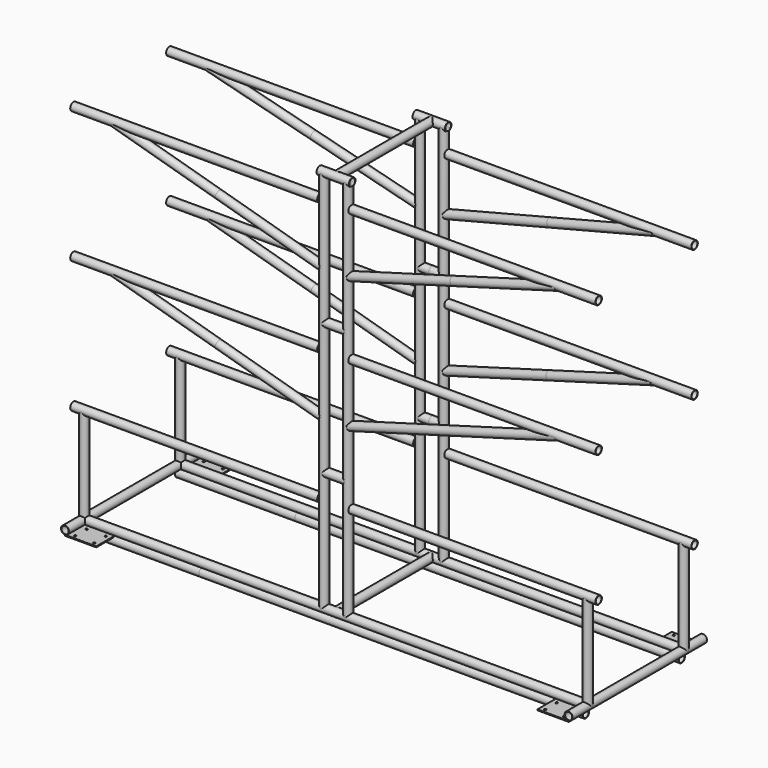
from build123d import *

# Parameters (mm, degrees)
F1_DEPTH       = 1600
F3_R           = 17
F4_DEPTH       = 50
F4_DEPTH_BACK  = 650
F5_DEPTH       = 50
F5_DEPTH_BACK  = 650
F7_R           = 17
F8_DEPTH       = 500
F8_DEPTH_BACK  = 1600
F10_W          = 130
F10_H          = 100
F10_R          = 4.5
F11_DEPTH      = 4
F14_R          = 17
F15_DEPTH      = 500
F15_DEPTH_BACK = 1600
F17_R          = 17
F18_DEPTH      = 500
F21_R          = 17
F22_DEPTH      = 530
F22_DEPTH_BACK = 500
F24_R          = 17
F25_DEPTH      = 530
F25_DEPTH_BACK = 500
F27_R          = 17
F28_DEPTH      = 450
F28_DEPTH_BACK = 450
F30_R          = 17
F31_DEPTH      = 450
F31_DEPTH_BACK = 450
F33_R          = 17
F34_DEPTH      = 50
F34_DEPTH_BACK = 50
F35_DEPTH      = 67.5
F35_DEPTH_BACK = 67.5
F37_R          = 17
F38_DEPTH      = 450
F38_DEPTH_BACK = 450
F40_R          = 17
F41_DEPTH      = 450
F41_DEPTH_BACK = 450
F45_R          = 17
F46_DEPTH      = 530
F46_DEPTH_BACK = 500
F48_R          = 17
F49_DEPTH      = 530
F49_DEPTH_BACK = 500
F51_R          = 17
F52_DEPTH      = 450
F52_DEPTH_BACK = 450
F54_R          = 17
F55_DEPTH      = 450
F55_DEPTH_BACK = 450
F57_R          = 17
F58_DEPTH      = 50
F58_DEPTH_BACK = 50
F59_DEPTH      = 67.5
F59_DEPTH_BACK = 67.5
F61_R          = 17
F62_DEPTH      = 450
F62_DEPTH_BACK = 450
F64_R          = 17
F65_DEPTH      = 450
F65_DEPTH_BACK = 450
F67_R          = 17
F68_DEPTH      = 200
F68_DEPTH_BACK = 200
F67_R_2        = 17.5
F70_R          = 17
F71_DEPTH      = 500
F72_R          = 15
F73_DEPTH      = 1020
F74_R          = 15
F75_DEPTH      = 1020
F76_R          = 15
F77_DEPTH      = 1020
F78_R          = 15
F79_DEPTH      = 1020
F80_R          = 15
F81_DEPTH      = 1020
F82_R          = 15
F83_DEPTH      = 1020
F84_R          = 15
F85_DEPTH      = 200
F86_R          = 15
F87_DEPTH      = 200
F88_R          = 15
F89_DEPTH      = 1020
F90_R          = 15
F91_DEPTH      = 1020
F92_R          = 15
F93_DEPTH      = 1020
F94_R          = 15
F95_DEPTH      = 1020
F96_R          = 15
F97_DEPTH      = 1020
F98_R          = 15
F99_DEPTH      = 1020
F100_R         = 15
F101_DEPTH     = 2300
F102_R         = 15
F103_DEPTH     = 2300
F104_R         = 15
F105_DEPTH     = 700
F106_R         = 15
F107_DEPTH     = 700


with BuildPart() as f1:
    # F0 (on Top) → F1 (new body)
    with BuildSketch(Plane.XY):
        with BuildLine():
            ThreePointArc((-25.1075440943, -100), (-42.1075440943, -83), (-59.1075440943, -100))
            ThreePointArc((-59.1075440943, -100), (-42.1075440943, -117), (-25.1075440943, -100))
        make_face()
    extrude(amount=F1_DEPTH)

    # F45 (on line) → F46 (join, two sides)
    with BuildSketch(Plane(origin=(-557.1075440943, 0, 0), x_dir=(0, -1, 0), z_dir=(-1, 0, 0))) as f46_sk:
        with Locations((100, 1500)):
            Circle(F45_R)
        with Locations((100, 950)):
            Circle(F45_R)
        with Locations((100, 400)):
            Circle(F45_R)
    extrude(amount=F46_DEPTH)
    extrude(f46_sk.sketch, amount=-F46_DEPTH_BACK)

    # F51 (on line) → F52 (join, two sides)
    with BuildSketch(Plane(origin=(-662.975364018, 0, 188.3452738687), x_dir=(0, -1, 0), z_dir=(-0.9619353575, 0, 0.2732770902))) as f52_sk:
        with Locations((100, 661.8477231125)):
            Circle(F51_R)
    extrude(amount=F52_DEPTH)
    extrude(f52_sk.sketch, amount=-F52_DEPTH_BACK)

    # F57 (on line) → F58 (join, two sides)
    with BuildSketch(Plane(origin=(7.8924559057, 0, 0), x_dir=(0, -1, 0), z_dir=(-1, 0, 0))) as f58_sk:
        with Locations((100, 1050)):
            Circle(F57_R)
        with Locations((100, 500)):
            Circle(F57_R)
    extrude(amount=F58_DEPTH)
    extrude(f58_sk.sketch, amount=-F58_DEPTH_BACK)

    # F61 (on line) → F62 (join, two sides)
    with BuildSketch(Plane(origin=(-787.0224706544, 0, 199.8620659412), x_dir=(0, -1, 0), z_dir=(-0.9692356631, 0, 0.2461345759))) as f62_sk:
        with Locations((100, 1225.2471397676)):
            Circle(F61_R)
    extrude(amount=F62_DEPTH)
    extrude(f62_sk.sketch, amount=-F62_DEPTH_BACK)


with BuildPart() as f1b:
    # F0 (on Top) → F1, piece 2 (new body)
    with BuildSketch(Plane.XY):
        with BuildLine():
            ThreePointArc((74.8924559057, -100), (57.8924559057, -83), (40.8924559057, -100))
            ThreePointArc((40.8924559057, -100), (57.8924559057, -117), (74.8924559057, -100))
        make_face()
    extrude(amount=F1_DEPTH)

    # F48 (on line) → F49 (join, two sides)
    with BuildSketch(Plane.YZ.offset(572.8924559057)) as f49_sk:
        with Locations((-100, 1500)):
            Circle(F48_R)
        with Locations((-100, 950)):
            Circle(F48_R)
        with Locations((-100, 400)):
            Circle(F48_R)
    extrude(amount=F49_DEPTH)
    extrude(f49_sk.sketch, amount=-F49_DEPTH_BACK)

    # F54 (on line) → F55 (join, two sides)
    with BuildSketch(Plane(origin=(677.581452806, 0, 192.4947309108), x_dir=(0, 1, 0), z_dir=(0.9619353575, 0, 0.2732770902))) as f55_sk:
        with Locations((-100, 657.5340683437)):
            Circle(F54_R)
    extrude(amount=F55_DEPTH)
    extrude(f55_sk.sketch, amount=-F55_DEPTH_BACK)

    # F64 (on line) → F65 (join, two sides)
    with BuildSketch(Plane(origin=(801.8510973168, 0, 203.6277525262), x_dir=(0, 1, 0), z_dir=(0.9692356631, 0, 0.2461345759))) as f65_sk:
        with Locations((-100, 1221.361927194)):
            Circle(F64_R)
    extrude(amount=F65_DEPTH)
    extrude(f65_sk.sketch, amount=-F65_DEPTH_BACK)


with BuildPart() as f1c:
    # F0 (on Top) → F1, piece 3 (new body)
    with BuildSketch(Plane.XY):
        with BuildLine():
            ThreePointArc((-25.1075440943, -600), (-42.1075440943, -583), (-59.1075440943, -600))
            ThreePointArc((-59.1075440943, -600), (-42.1075440943, -617), (-25.1075440943, -600))
        make_face()
    extrude(amount=F1_DEPTH)

    # F24 (on line) → F25 (join, two sides)
    with BuildSketch(Plane(origin=(-557.1075440943, 0, 0), x_dir=(0, -1, 0), z_dir=(-1, 0, 0))) as f25_sk:
        with Locations((600, 1500)):
            Circle(F24_R)
        with Locations((600, 950)):
            Circle(F24_R)
        with Locations((600, 400)):
            Circle(F24_R)
    extrude(amount=F25_DEPTH)
    extrude(f25_sk.sketch, amount=-F25_DEPTH_BACK)

    # F30 (on line) → F31 (join, two sides)
    with BuildSketch(Plane(origin=(-807.5565565141, 0, 229.4194762824), x_dir=(0, -1, 0), z_dir=(-0.9619353575, 0, 0.2732770902))) as f31_sk:
        with Locations((600, 1190.9121697279)):
            Circle(F30_R)
    extrude(amount=F31_DEPTH)
    extrude(f31_sk.sketch, amount=-F31_DEPTH_BACK)

    # F40 (on line) → F41 (join, two sides)
    with BuildSketch(Plane(origin=(-662.975364018, 0, 188.3452738687), x_dir=(0, -1, 0), z_dir=(-0.9619353575, 0, 0.2732770902))) as f41_sk:
        with Locations((600, 661.8477231125)):
            Circle(F40_R)
    extrude(amount=F41_DEPTH)
    extrude(f41_sk.sketch, amount=-F41_DEPTH_BACK)


with BuildPart() as f1d:
    # F0 (on Top) → F1, piece 4 (new body)
    with BuildSketch(Plane.XY):
        with BuildLine():
            ThreePointArc((74.8924559057, -600), (57.8924559057, -583), (40.8924559057, -600))
            ThreePointArc((40.8924559057, -600), (57.8924559057, -617), (74.8924559057, -600))
        make_face()
    extrude(amount=F1_DEPTH)

    # F21 (on line) → F22 (join, two sides)
    with BuildSketch(Plane.YZ.offset(572.8924559057)) as f22_sk:
        with Locations((-600, 1500)):
            Circle(F21_R)
        with Locations((-600, 950)):
            Circle(F21_R)
        with Locations((-600, 400)):
            Circle(F21_R)
    extrude(amount=F22_DEPTH)
    extrude(f22_sk.sketch, amount=-F22_DEPTH_BACK)

    # F27 (on line) → F28 (join, two sides)
    with BuildSketch(Plane(origin=(822.1626453021, 0, 233.5689333245), x_dir=(0, 1, 0), z_dir=(0.9619353575, 0, 0.2732770902))) as f28_sk:
        with Locations((-600, 1186.5985149591)):
            Circle(F27_R)
    extrude(amount=F28_DEPTH)
    extrude(f28_sk.sketch, amount=-F28_DEPTH_BACK)


with BuildPart() as f4:
    # F3 (on line) → F4 (new body, two sides)
    with BuildSketch(Plane(origin=(0, -50, 0), x_dir=(-1, 0, 0), z_dir=(0, 1, 0))) as f4_sk:
        with Locations((1042.1075440943, 0)):
            Circle(F3_R)
    extrude(amount=F4_DEPTH)
    extrude(f4_sk.sketch, amount=-F4_DEPTH_BACK)


with BuildPart() as f4b:
    # F3 (on line) → F4, piece 2 (new body, two sides)
    with BuildSketch(Plane(origin=(0, -50, 0), x_dir=(-1, 0, 0), z_dir=(0, 1, 0))) as f4_2_sk:
        with Locations((-1057.8924559057, 0)):
            Circle(F3_R)
    extrude(amount=F4_DEPTH)
    extrude(f4_2_sk.sketch, amount=-F4_DEPTH_BACK)


with BuildPart() as f5:
    # F3 (on line) → F5 (new body, two sides)
    with BuildSketch(Plane(origin=(0, -50, 0), x_dir=(-1, 0, 0), z_dir=(0, 1, 0))) as f5_sk:
        with Locations((1042.1075440943, 0)):
            Circle(F3_R)
    extrude(amount=F5_DEPTH)
    extrude(f5_sk.sketch, amount=-F5_DEPTH_BACK)


with BuildPart() as f5b:
    # F3 (on line) → F5, piece 2 (new body, two sides)
    with BuildSketch(Plane(origin=(0, -50, 0), x_dir=(-1, 0, 0), z_dir=(0, 1, 0))) as f5_2_sk:
        with Locations((-1057.8924559057, 0)):
            Circle(F3_R)
    extrude(amount=F5_DEPTH)
    extrude(f5_2_sk.sketch, amount=-F5_DEPTH_BACK)


with BuildPart() as f8:
    # F7 (on line) → F8 (new body, two sides)
    with BuildSketch(Plane.YZ.offset(-550.6075440943)) as f8_sk:
        with Locations((-100, 0)):
            Circle(F7_R)
    extrude(amount=-F8_DEPTH)
    extrude(f8_sk.sketch, amount=F8_DEPTH_BACK)


with BuildPart() as f8b:
    # F7 (on line) → F8, piece 2 (new body, two sides)
    with BuildSketch(Plane.YZ.offset(-550.6075440943)) as f8_2_sk:
        with Locations((-600, 0)):
            Circle(F7_R)
    extrude(amount=-F8_DEPTH)
    extrude(f8_2_sk.sketch, amount=F8_DEPTH_BACK)


with BuildPart() as f11:
    # F10 (on offset) → F11 (new body)
    with BuildSketch(Plane.XY.offset(-17.5)):
        with Locations((-977.1075440943, -650)):
            Rectangle(F10_W, F10_H)
        with Locations((-1012.1075440943, -685)):
            Circle(F10_R, mode=Mode.SUBTRACT)
        with Locations((-932.1075440943, -685)):
            Circle(F10_R, mode=Mode.SUBTRACT)
        with Locations((-1012.1075440943, -625)):
            Circle(F10_R, mode=Mode.SUBTRACT)
        with Locations((-932.1075440943, -625)):
            Circle(F10_R, mode=Mode.SUBTRACT)
    extrude(amount=-F11_DEPTH)


with BuildPart() as f11b:
    # F10 (on offset) → F11, piece 2 (new body)
    with BuildSketch(Plane.XY.offset(-17.5)):
        with Locations((-977.1075440943, -50)):
            Rectangle(F10_W, F10_H)
        with Locations((-1012.1075440943, -75)):
            Circle(F10_R, mode=Mode.SUBTRACT)
        with Locations((-932.1075440943, -75)):
            Circle(F10_R, mode=Mode.SUBTRACT)
        with Locations((-1012.1075440943, -15)):
            Circle(F10_R, mode=Mode.SUBTRACT)
        with Locations((-932.1075440943, -15)):
            Circle(F10_R, mode=Mode.SUBTRACT)
    extrude(amount=-F11_DEPTH)


with BuildPart() as f11c:
    # F10 (on offset) → F11, piece 3 (new body)
    with BuildSketch(Plane.XY.offset(-17.5)):
        with Locations((992.8924559057, -650)):
            Rectangle(F10_W, F10_H)
        with Locations((947.8924559057, -685)):
            Circle(F10_R, mode=Mode.SUBTRACT)
        with Locations((1027.8924559057, -685)):
            Circle(F10_R, mode=Mode.SUBTRACT)
        with Locations((947.8924559057, -625)):
            Circle(F10_R, mode=Mode.SUBTRACT)
        with Locations((1027.8924559057, -625)):
            Circle(F10_R, mode=Mode.SUBTRACT)
    extrude(amount=-F11_DEPTH)


with BuildPart() as f11d:
    # F10 (on offset) → F11, piece 4 (new body)
    with BuildSketch(Plane.XY.offset(-17.5)):
        with Locations((992.8924559057, -50)):
            Rectangle(F10_W, F10_H)
        with Locations((947.8924559057, -75)):
            Circle(F10_R, mode=Mode.SUBTRACT)
        with Locations((1027.8924559057, -75)):
            Circle(F10_R, mode=Mode.SUBTRACT)
        with Locations((947.8924559057, -15)):
            Circle(F10_R, mode=Mode.SUBTRACT)
        with Locations((1027.8924559057, -15)):
            Circle(F10_R, mode=Mode.SUBTRACT)
    extrude(amount=-F11_DEPTH)


with BuildPart() as f15:
    # F14 (on line) → F15 (new body, two sides)
    with BuildSketch(Plane.YZ.offset(-550.6075440943)) as f15_sk:
        with Locations((-100, -35)):
            Circle(F14_R)
    extrude(amount=-F15_DEPTH)
    extrude(f15_sk.sketch, amount=F15_DEPTH_BACK)


with BuildPart() as f15b:
    # F14 (on line) → F15, piece 2 (new body, two sides)
    with BuildSketch(Plane.YZ.offset(-550.6075440943)) as f15_2_sk:
        with Locations((-600, -35)):
            Circle(F14_R)
    extrude(amount=-F15_DEPTH)
    extrude(f15_2_sk.sketch, amount=F15_DEPTH_BACK)


with BuildPart() as f18:
    # F17 (on face) → F18 (new body)
    with BuildSketch(Plane(origin=(0, -600, 0), x_dir=(-1, 0, 0), z_dir=(0, 1, 0))):
        with Locations((-7.8924559057, 0)):
            Circle(F17_R)
    extrude(amount=F18_DEPTH)


with BuildPart() as f34:
    # F33 (on line) → F34 (new body, two sides)
    with BuildSketch(Plane.YZ.offset(7.8924559057)) as f34_sk:
        with Locations((-600, 1050)):
            Circle(F33_R)
    extrude(amount=F34_DEPTH)
    extrude(f34_sk.sketch, amount=-F34_DEPTH_BACK)


with BuildPart() as f34b:
    # F33 (on line) → F34, piece 2 (new body, two sides)
    with BuildSketch(Plane.YZ.offset(7.8924559057)) as f34_2_sk:
        with Locations((-600, 500)):
            Circle(F33_R)
    extrude(amount=F34_DEPTH)
    extrude(f34_2_sk.sketch, amount=-F34_DEPTH_BACK)


with BuildPart() as f35:
    # F33 (on line) → F35 (new body, two sides)
    with BuildSketch(Plane.YZ.offset(7.8924559057)) as f35_sk:
        with Locations((-600, 1600)):
            Circle(F33_R)
    extrude(amount=F35_DEPTH)
    extrude(f35_sk.sketch, amount=-F35_DEPTH_BACK)


with BuildPart() as f38:
    # F37 (on line) → F38 (new body, two sides)
    with BuildSketch(Plane(origin=(677.581452806, 0, 192.4947309108), x_dir=(0, 1, 0), z_dir=(0.9619353575, 0, 0.2732770902))) as f38_sk:
        with Locations((-600, 657.5340683437)):
            Circle(F37_R)
    extrude(amount=F38_DEPTH)
    extrude(f38_sk.sketch, amount=-F38_DEPTH_BACK)


with BuildPart() as f59:
    # F57 (on line) → F59 (new body, two sides)
    with BuildSketch(Plane(origin=(7.8924559057, 0, 0), x_dir=(0, -1, 0), z_dir=(-1, 0, 0))) as f59_sk:
        with Locations((100, 1600)):
            Circle(F57_R)
    extrude(amount=F59_DEPTH)
    extrude(f59_sk.sketch, amount=-F59_DEPTH_BACK)


with BuildPart() as f68:
    # F67 (on line) → F68 (new body, two sides)
    with BuildSketch(Plane(origin=(0, 0, 200), x_dir=(1, 0, 0), z_dir=(0, 0, -1))) as f68_sk:
        with Locations((-1042.1075440943, 600)):
            Circle(F67_R)
    extrude(amount=F68_DEPTH)
    extrude(f68_sk.sketch, amount=-F68_DEPTH_BACK)


with BuildPart() as f68b:
    # F67 (on line) → F68, piece 2 (new body, two sides)
    with BuildSketch(Plane(origin=(0, 0, 200), x_dir=(1, 0, 0), z_dir=(0, 0, -1))) as f68_2_sk:
        with Locations((-1042.1075440943, 100)):
            Circle(F67_R)
    extrude(amount=F68_DEPTH)
    extrude(f68_2_sk.sketch, amount=-F68_DEPTH_BACK)


with BuildPart() as f68c:
    # F67 (on line) → F68, piece 3 (new body, two sides)
    with BuildSketch(Plane(origin=(0, 0, 200), x_dir=(1, 0, 0), z_dir=(0, 0, -1))) as f68_3_sk:
        with Locations((1057.8924559057, 600)):
            Circle(F67_R_2)
    extrude(amount=F68_DEPTH)
    extrude(f68_3_sk.sketch, amount=-F68_DEPTH_BACK)


with BuildPart() as f68d:
    # F67 (on line) → F68, piece 4 (new body, two sides)
    with BuildSketch(Plane(origin=(0, 0, 200), x_dir=(1, 0, 0), z_dir=(0, 0, -1))) as f68_4_sk:
        with Locations((1057.8924559057, 100)):
            Circle(F67_R_2)
    extrude(amount=F68_DEPTH)
    extrude(f68_4_sk.sketch, amount=-F68_DEPTH_BACK)


with BuildPart() as f71:
    # F70 (on face) → F71 (new body)
    with BuildSketch(Plane.XZ.offset(600)):
        with Locations((7.8924559057, 1600)):
            Circle(F70_R)
    extrude(amount=-F71_DEPTH)


with BuildPart() as f73_tool:
    # F72 (on face) → F73 (new body)
    with BuildSketch(Plane.YZ.offset(1102.8924559057)):
        with Locations((-600, 400)):
            Circle(F72_R)
    extrude(amount=-F73_DEPTH)


with BuildPart() as f1d_1:
    add(f1d.part)

    # F73: cut by f73_tool
    add(f73_tool.part, mode=Mode.SUBTRACT)


with BuildPart() as f68c_1:
    add(f68c.part)

    # F73: cut by f73_tool
    add(f73_tool.part, mode=Mode.SUBTRACT)


with BuildPart() as f75_tool:
    # F74 (on face) → F75 (new body)
    with BuildSketch(Plane.YZ.offset(1102.8924559057)):
        with Locations((-100, 400)):
            Circle(F74_R)
    extrude(amount=-F75_DEPTH)


with BuildPart() as f1b_1:
    add(f1b.part)

    # F75: cut by f75_tool
    add(f75_tool.part, mode=Mode.SUBTRACT)

    # F76 (on face) → F77 (cut)
    with BuildSketch(Plane.YZ.offset(1102.8924559057)):
        with Locations((-100, 950)):
            Circle(F76_R)
    extrude(amount=-F77_DEPTH, mode=Mode.SUBTRACT)

    # F82 (on face) → F83 (cut)
    with BuildSketch(Plane.YZ.offset(1102.8924559057)):
        with Locations((-100, 1500)):
            Circle(F82_R)
    extrude(amount=-F83_DEPTH, mode=Mode.SUBTRACT)


with BuildPart() as f68d_1:
    add(f68d.part)

    # F75: cut by f75_tool
    add(f75_tool.part, mode=Mode.SUBTRACT)


with BuildPart() as f79_tool:
    # F78 (on face) → F79 (new body)
    with BuildSketch(Plane.YZ.offset(1102.8924559057)):
        with Locations((-600, 950)):
            Circle(F78_R)
    extrude(amount=-F79_DEPTH)


with BuildPart() as f1d_2:
    add(f1d_1.part)

    # F79: cut by f79_tool
    add(f79_tool.part, mode=Mode.SUBTRACT)

    # F80 (on face) → F81 (cut)
    with BuildSketch(Plane.YZ.offset(1102.8924559057)):
        with Locations((-600, 1500)):
            Circle(F80_R)
    extrude(amount=-F81_DEPTH, mode=Mode.SUBTRACT)


with BuildPart() as f38_1:
    add(f38.part)

    # F79: cut by f79_tool
    add(f79_tool.part, mode=Mode.SUBTRACT)


with BuildPart() as f85_tool:
    # F84 (on face) → F85 (new body)
    with BuildSketch(Plane.YZ.offset(75.3924559057)):
        with Locations((-600, 1600)):
            Circle(F84_R)
    extrude(amount=-F85_DEPTH)


with BuildPart() as f1c_1:
    add(f1c.part)

    # F85: cut by f85_tool
    add(f85_tool.part, mode=Mode.SUBTRACT)

    # F90 (on face) → F91 (cut)
    with BuildSketch(Plane(origin=(-1087.1075440943, 0, 0), x_dir=(0, -1, 0), z_dir=(-1, 0, 0))):
        with Locations((600, 1500)):
            Circle(F90_R)
    extrude(amount=-F91_DEPTH, mode=Mode.SUBTRACT)

    # F94 (on face) → F95 (cut)
    with BuildSketch(Plane(origin=(-1087.1075440943, 0, 0), x_dir=(0, -1, 0), z_dir=(-1, 0, 0))):
        with Locations((600, 950)):
            Circle(F94_R)
    extrude(amount=-F95_DEPTH, mode=Mode.SUBTRACT)


with BuildPart() as f1d_3:
    add(f1d_2.part)

    # F85: cut by f85_tool
    add(f85_tool.part, mode=Mode.SUBTRACT)


with BuildPart() as f35_1:
    add(f35.part)

    # F85: cut by f85_tool
    add(f85_tool.part, mode=Mode.SUBTRACT)


with BuildPart() as f71_1:
    add(f71.part)

    # F85: cut by f85_tool
    add(f85_tool.part, mode=Mode.SUBTRACT)


with BuildPart() as f87_tool:
    # F86 (on face) → F87 (new body)
    with BuildSketch(Plane.YZ.offset(75.3924559057)):
        with Locations((-100, 1600)):
            Circle(F86_R)
    extrude(amount=-F87_DEPTH)


with BuildPart() as f1_1:
    add(f1.part)

    # F87: cut by f87_tool
    add(f87_tool.part, mode=Mode.SUBTRACT)

    # F88 (on face) → F89 (cut)
    with BuildSketch(Plane(origin=(-1087.1075440943, 0, 0), x_dir=(0, -1, 0), z_dir=(-1, 0, 0))):
        with Locations((100, 1500)):
            Circle(F88_R)
    extrude(amount=-F89_DEPTH, mode=Mode.SUBTRACT)

    # F92 (on face) → F93 (cut)
    with BuildSketch(Plane(origin=(-1087.1075440943, 0, 0), x_dir=(0, -1, 0), z_dir=(-1, 0, 0))):
        with Locations((100, 950)):
            Circle(F92_R)
    extrude(amount=-F93_DEPTH, mode=Mode.SUBTRACT)


with BuildPart() as f1b_2:
    add(f1b_1.part)

    # F87: cut by f87_tool
    add(f87_tool.part, mode=Mode.SUBTRACT)


with BuildPart() as f59_1:
    add(f59.part)

    # F87: cut by f87_tool
    add(f87_tool.part, mode=Mode.SUBTRACT)


with BuildPart() as f71_2:
    add(f71_1.part)

    # F87: cut by f87_tool
    add(f87_tool.part, mode=Mode.SUBTRACT)


with BuildPart() as f97_tool:
    # F96 (on face) → F97 (new body)
    with BuildSketch(Plane(origin=(-1087.1075440943, 0, 0), x_dir=(0, -1, 0), z_dir=(-1, 0, 0))):
        with Locations((100, 400)):
            Circle(F96_R)
    extrude(amount=-F97_DEPTH)


with BuildPart() as f1_2:
    add(f1_1.part)

    # F97: cut by f97_tool
    add(f97_tool.part, mode=Mode.SUBTRACT)


with BuildPart() as f68b_1:
    add(f68b.part)

    # F97: cut by f97_tool
    add(f97_tool.part, mode=Mode.SUBTRACT)


with BuildPart() as f99_tool:
    # F98 (on face) → F99 (new body)
    with BuildSketch(Plane(origin=(-1087.1075440943, 0, 0), x_dir=(0, -1, 0), z_dir=(-1, 0, 0))):
        with Locations((600, 400)):
            Circle(F98_R)
    extrude(amount=-F99_DEPTH)


with BuildPart() as f1c_2:
    add(f1c_1.part)

    # F99: cut by f99_tool
    add(f99_tool.part, mode=Mode.SUBTRACT)


with BuildPart() as f68_1:
    add(f68.part)

    # F99: cut by f99_tool
    add(f99_tool.part, mode=Mode.SUBTRACT)


with BuildPart() as f101_tool:
    # F100 (on face) → F101 (new body)
    with BuildSketch(Plane(origin=(-1050.6075440943, 0, 0), x_dir=(0, -1, 0), z_dir=(-1, 0, 0))):
        with Locations((600, -35)):
            Circle(F100_R)
    extrude(amount=-F101_DEPTH)


with BuildPart() as f11_1:
    add(f11.part)

    # F101: cut by f101_tool
    add(f101_tool.part, mode=Mode.SUBTRACT)


with BuildPart() as f11c_1:
    add(f11c.part)

    # F101: cut by f101_tool
    add(f101_tool.part, mode=Mode.SUBTRACT)


with BuildPart() as f15b_1:
    add(f15b.part)

    # F101: cut by f101_tool
    add(f101_tool.part, mode=Mode.SUBTRACT)


with BuildPart() as f103_tool:
    # F102 (on face) → F103 (new body)
    with BuildSketch(Plane(origin=(-1050.6075440943, 0, 0), x_dir=(0, -1, 0), z_dir=(-1, 0, 0))):
        with Locations((100, -35)):
            Circle(F102_R)
    extrude(amount=-F103_DEPTH)


with BuildPart() as f11b_1:
    add(f11b.part)

    # F103: cut by f103_tool
    add(f103_tool.part, mode=Mode.SUBTRACT)


with BuildPart() as f11d_1:
    add(f11d.part)

    # F103: cut by f103_tool
    add(f103_tool.part, mode=Mode.SUBTRACT)


with BuildPart() as f15_1:
    add(f15.part)

    # F103: cut by f103_tool
    add(f103_tool.part, mode=Mode.SUBTRACT)


with BuildPart() as f105_tool:
    # F104 (on face) → F105 (new body)
    with BuildSketch(Plane.XZ.offset(700)):
        with Locations((-1042.1075440943, 0)):
            Circle(F104_R)
    extrude(amount=-F105_DEPTH)


with BuildPart() as f4_1:
    add(f4.part)

    # F105: cut by f105_tool
    add(f105_tool.part, mode=Mode.SUBTRACT)


with BuildPart() as f5_1:
    add(f5.part)

    # F105: cut by f105_tool
    add(f105_tool.part, mode=Mode.SUBTRACT)


with BuildPart() as f8_1:
    add(f8.part)

    # F105: cut by f105_tool
    add(f105_tool.part, mode=Mode.SUBTRACT)


with BuildPart() as f8b_1:
    add(f8b.part)

    # F105: cut by f105_tool
    add(f105_tool.part, mode=Mode.SUBTRACT)


with BuildPart() as f68_2:
    add(f68_1.part)

    # F105: cut by f105_tool
    add(f105_tool.part, mode=Mode.SUBTRACT)


with BuildPart() as f68b_2:
    add(f68b_1.part)

    # F105: cut by f105_tool
    add(f105_tool.part, mode=Mode.SUBTRACT)


with BuildPart() as f107_tool:
    # F106 (on face) → F107 (new body)
    with BuildSketch(Plane.XZ.offset(700)):
        with Locations((1057.8924559057, 0)):
            Circle(F106_R)
    extrude(amount=-F107_DEPTH)


with BuildPart() as f4b_1:
    add(f4b.part)

    # F107: cut by f107_tool
    add(f107_tool.part, mode=Mode.SUBTRACT)


with BuildPart() as f5b_1:
    add(f5b.part)

    # F107: cut by f107_tool
    add(f107_tool.part, mode=Mode.SUBTRACT)


with BuildPart() as f8_2:
    add(f8_1.part)

    # F107: cut by f107_tool
    add(f107_tool.part, mode=Mode.SUBTRACT)


with BuildPart() as f8b_2:
    add(f8b_1.part)

    # F107: cut by f107_tool
    add(f107_tool.part, mode=Mode.SUBTRACT)


with BuildPart() as f68c_2:
    add(f68c_1.part)

    # F107: cut by f107_tool
    add(f107_tool.part, mode=Mode.SUBTRACT)


with BuildPart() as f68d_2:
    add(f68d_1.part)

    # F107: cut by f107_tool
    add(f107_tool.part, mode=Mode.SUBTRACT)


solid = Compound([f18.part, f34.part, f34b.part, f38_1.part, f1d_3.part, f35_1.part, f1b_2.part, f59_1.part, f71_2.part, f1_2.part, f1c_2.part, f11_1.part, f11c_1.part, f15b_1.part, f11b_1.part, f11d_1.part, f15_1.part, f4_1.part, f5_1.part, f68_2.part, f68b_2.part, f4b_1.part, f5b_1.part, f8_2.part, f8b_2.part, f68c_2.part, f68d_2.part])
